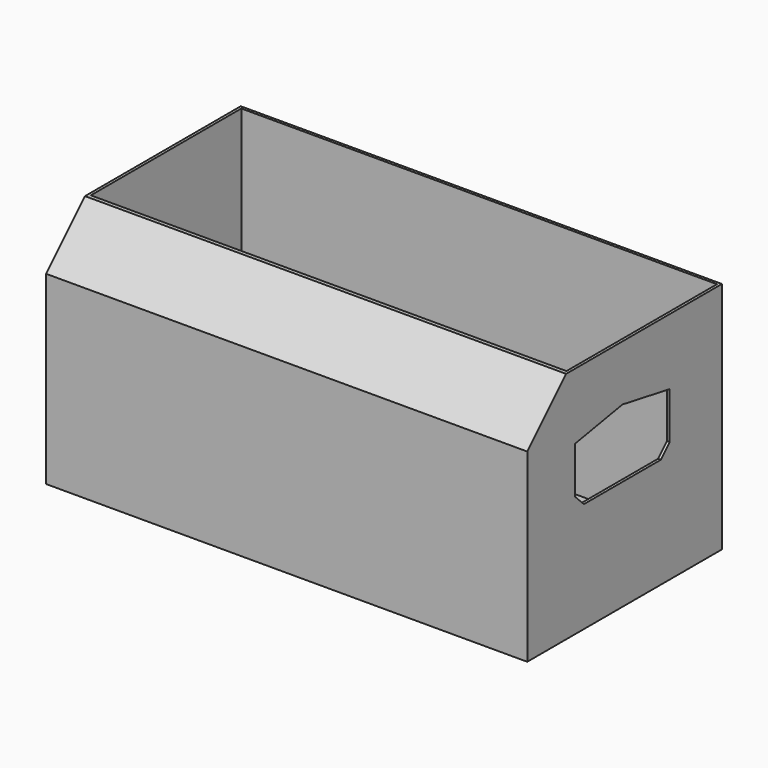
from build123d import *

# Parameters (mm, degrees)
F0_W        = 175
F0_H        = 88.5
F1_DEPTH    = 85
F2_SIZE     = 17.678
F3_T        = -1
F4_W        = 43
F4_H        = 25
F5_DEPTH    = 2
F6_T1_DEPTH = 1
F7_SIZE     = 4


# Not quite as in the source:
# - a fillet or chamfer that OpenCascade refuses, or shapes differently, is made with other operations: its cross-section is extruded or revolved along the edge and cut away or added


with BuildPart() as f1:
    # F0 (on Top) → F1 (new body)
    with BuildSketch(Plane.XY):
        with Locations((87.5, -44.25)):
            Rectangle(F0_W, F0_H)
    extrude(amount=F1_DEPTH)

    # F2
    f2_edges = [f1.edges().sort_by_distance(p)[0] for p in [
        (87.5, -88.5, 85),
    ]]
    chamfer(f2_edges, length=F2_SIZE)

    # F3
    f3_openings = [f1.faces().sort_by_distance(p)[0] for p in [
        (87.5, -35.411, 85),
    ]]
    offset(amount=F3_T, openings=f3_openings, kind=Kind.INTERSECTION)

    # F4 (on face) → F5 (cut)
    with BuildSketch(Plane.YZ.offset(175)):
        with Locations((-45.25, 52.5)):
            Rectangle(F4_W, F4_H)
    extrude(amount=-F5_DEPTH, mode=Mode.SUBTRACT)

    # F6: chamfer of 4 x 22.6851272785 on 2 edges, made by hand

    # F6_s2 → F6_t1 (join)
    with BuildSketch(Plane.YZ.offset(174)):
        Polygon((-66.75, 61), (-44.0648727215, 65), (-66.75, 65), align=None)
        Polygon((-23.75, 61), (-46.4351272785, 65), (-23.75, 65), align=None)
    extrude(amount=F6_T1_DEPTH)

    # F7
    f7_edges = [f1.edges().sort_by_distance(p)[0] for p in [
        (174.5, -66.75, 40),
        (174.5, -23.75, 40),
    ]]
    chamfer(f7_edges, length=F7_SIZE)


solid = f1.part
